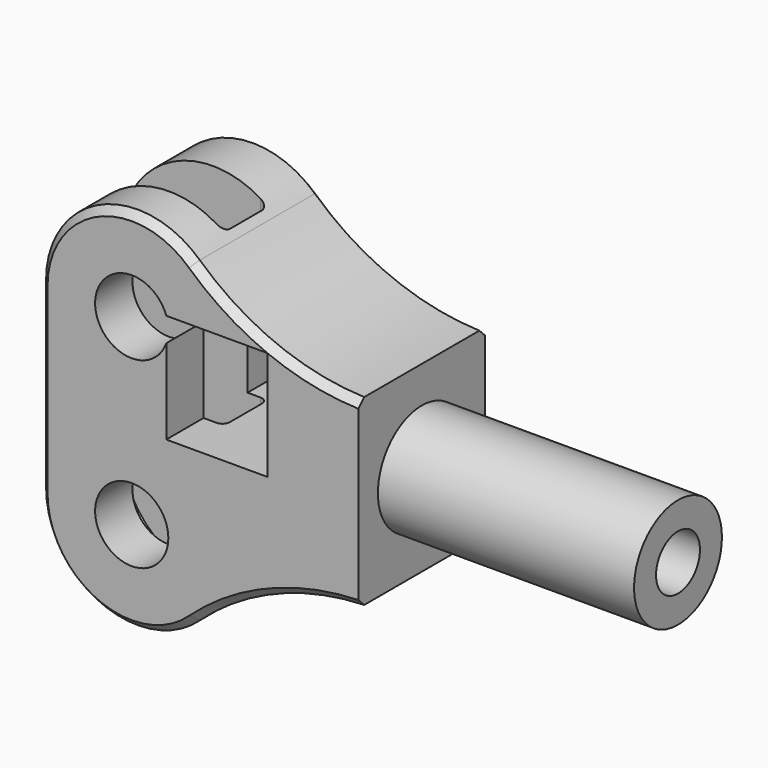
from build123d import *

# Parameters (mm, degrees)
F9_R        = 10
F9_W        = 36.9291573763
F9_H        = 50
F0_DEPTH    = 43.3197319508
F1_W        = 15
F1_H        = 36.1227724802
F1_H_2      = 37.2449353439
F1_H_3      = 50
F11_DEPTH   = 40
F2_T4_DEPTH = 43.3197319508
F2_T9_DEPTH = 43.3197319508
F12_R       = 15
F3_DEPTH    = 70
F4_D        = 15
F4_DEPTH    = 35
F4_TIP      = 4.5064546427
F5_SIZE     = 2
F6_R        = 2
F8_DEPTH    = 66.8339151889


# Not quite as in the source:
# - a fillet or chamfer that OpenCascade refuses, or shapes differently, is made with other operations: its cross-section is extruded or revolved along the edge and cut away or added


with BuildPart() as f0:
    # F9 (on Front) → F0 (new body)
    with BuildSketch(Plane.XZ):
        with BuildLine():
            Line((0, 50), (0, 0))
            ThreePointArc((0, 0), (25, -25), (50, 0))
            Line((50, 0), (50, 50))
            ThreePointArc((50, 50), (25, 75), (0, 50))
        make_face()
        with Locations((25, 0)):
            Circle(F9_R, mode=Mode.SUBTRACT)
        with Locations((25, 50)):
            Circle(F9_R, mode=Mode.SUBTRACT)
        with Locations((68.4645786881, 25)):
            Rectangle(F9_W, F9_H)
    extrude(amount=F0_DEPTH)

    # F1 (on face) → F11 (cut)
    with BuildSketch(Plane(origin=(0, 0, 0), x_dir=(0, -1, 0), z_dir=(-1, 0, 0))):
        with Locations((23.0782711878, 68.0613862401)):
            Rectangle(F1_W, F1_H)
        with Locations((23.0782711878, -18.6224676719)):
            Rectangle(F1_W, F1_H_2)
        with Locations((23.0782711878, 25)):
            Rectangle(F1_W, F1_H_3)
    extrude(amount=-F11_DEPTH, mode=Mode.SUBTRACT)

    # F2: fillet of radius 70 on 2 edges, made by hand


with BuildPart() as f2_tool2:
    # F2_s3 → F2_t4 (new body)
    with BuildSketch(Plane.XZ):
        with BuildLine():
            ThreePointArc((41.9124921282, 68.4105298721), (62.7704674486, 55.169784882), (86.9291440051, 49.9996002235))
            Line((86.9291440051, 49.9996002235), (86.6951432376, 43.0033758404))
            ThreePointArc((86.6951432376, 43.0033758404), (68.4645720025, 42.9998634315), (50, 42.9998634315))
            Line((50, 42.9998634315), (42.9998634315, 50))
            ThreePointArc((42.9998634315, 50), (41.4800309388, 57.2390374918), (37.1768261731, 63.2553984539))
            Line((37.1768261731, 63.2553984539), (41.9124921282, 68.4105298721))
        make_face()
    extrude(amount=F2_T4_DEPTH)

    split(bisect_by=Plane.YZ.offset(40), keep=Keep.TOP)


with BuildPart() as f0_1:
    add(f0.part)

    # F2_t1: union F2_tool2
    add(f2_tool2.part)


with BuildPart() as f2_tool7:
    # F2_s8 → F2_t9 (new body)
    with BuildSketch(Plane.XZ):
        with BuildLine():
            ThreePointArc((41.9124921282, -18.4105298721), (62.7704674486, -5.169784882), (86.9291440051, 0.0003997765))
            Line((86.9291440051, 0.0003997765), (86.6951432376, 6.9966241596))
            ThreePointArc((86.6951432376, 6.9966241596), (68.4645720025, 7.0001365685), (50, 7.0001365685))
            Line((50, 7.0001365685), (42.9998634315, 0))
            ThreePointArc((42.9998634315, 0), (41.4800309388, -7.2390374918), (37.1768261731, -13.2553984539))
            Line((37.1768261731, -13.2553984539), (41.9124921282, -18.4105298721))
        make_face()
    extrude(amount=F2_T9_DEPTH)

    split(bisect_by=Plane.YZ.offset(40), keep=Keep.TOP)


with BuildPart() as f0_2:
    add(f0_1.part)

    # F2_t6: union F2_tool7
    add(f2_tool7.part)

    # F12 (on face) → F3 (join)
    with BuildSketch(Plane.YZ.offset(86.9291573763)):
        with Locations((-21.6598659754, 25)):
            Circle(F12_R)
    extrude(amount=F3_DEPTH)

    # F4
    with Locations(Plane.YZ.offset(156.9291573763)):
        with Locations((-21.6598659754, 25)):
            Hole(F4_D / 2, depth=F4_DEPTH)
            with Locations((0, 0, -(F4_DEPTH + F4_TIP / 2))):  # 118° drill point
                Cone(0, F4_D / 2, F4_TIP, mode=Mode.SUBTRACT)

    # F5
    f5_edges = [f0_2.edges().sort_by_distance(p)[0] for p in [
        (0, 0, 25),
        (15.001227, 0, 72.913414),
        (15.001227, 0, -22.913414),
        (62.821136, 0, -5.149086),
        (62.821136, 0, 55.149086),
        (0, -43.319732, 25),
        (15.001227, -43.319732, 72.913414),
        (62.821136, -43.319732, 55.149086),
        (15.001227, -43.319732, -22.913414),
        (62.821136, -43.319732, -5.149086),
        (86.92319, 0, 0),
        (86.92319, 0, 50),
        (86.92319, -43.319732, 0),
        (86.92319, -43.319732, 50),
    ]]
    chamfer(f5_edges, length=F5_SIZE)

    # F6
    f6_edges = [f0_2.edges().sort_by_distance(p)[0] for p in [
        (40, -30.578271, 25),
        (40, -15.578271, 25),
    ]]
    fillet(f6_edges, radius=F6_R)

    # F7 (on face) → F8 (cut)
    with BuildSketch(Plane.XZ.offset(43.3197319508)):
        with BuildLine():
            Line((62.0436161135, 53.3062600899), (34.4376185671, 53.3062600899))
            ThreePointArc((34.4376185671, 53.3062600899), (34.8584021441, 51.6768742244), (35, 50))
            ThreePointArc((35, 50), (34.8584021441, 48.3231257756), (34.4376185671, 46.6937399101))
            Line((34.4376185671, 46.6937399101), (34.4376185671, 23.5226601362))
            Line((34.4376185671, 23.5226601362), (62.0445043538, 23.5226601362))
            Line((62.0445043538, 23.5226601362), (62.0445043538, 53.3058972942))
            ThreePointArc((62.0445043538, 53.3058972942), (62.044060233, 53.3060786906), (62.0436161135, 53.3062600899))
        make_face()
    extrude(amount=-F8_DEPTH, mode=Mode.SUBTRACT)


solid = f0_2.part
